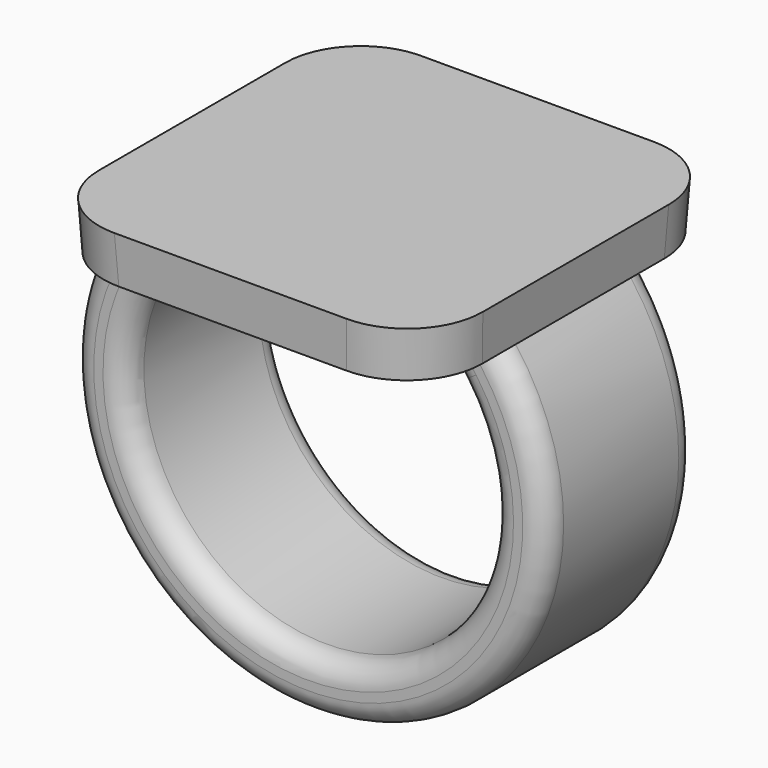
from build123d import *

# Parameters (mm, degrees)
F0_W          = 25.4
F0_H          = 25.4
F1_DEPTH      = 3.175
F1_TAPER      = -3
F3_W          = 5.08
F3_H          = 12.7
F6_DEPTH      = 6.35
F6_DEPTH_BACK = 6.35
F7_R          = 5.08
F8_R          = 1.524


with BuildPart() as f1:
    # F0 (on Top) → F1 (new body)
    with BuildSketch(Plane.XY):
        Rectangle(F0_W, F0_H)
    extrude(amount=F1_DEPTH, taper=F1_TAPER)

    # F4: sweep along a path in F2
    with BuildLine(Plane.XZ) as f4_path:
        ThreePointArc((-10.16, 0), (0, -23.5582897328), (10.16, 0))
    # F3 (on face) → F4 (sweep)
    with BuildSketch(Plane(origin=(0, 0, 0), x_dir=(1, 0, 0), z_dir=(0, 0, -1))):
        with Locations((-10.16, 0)):
            Rectangle(F3_W, F3_H)
    sweep(path=f4_path.line)

    # F5 (on Front) → F6 (join, two sides)
    with BuildSketch(Plane.XZ) as f6_sk:
        with BuildLine():
            Line((10.0130578512, -2.535746045), (10.16, 0))
            Line((10.16, 0), (7.62, 0))
            ThreePointArc((7.62, 0), (8.9072265211, -1.1822790439), (10.0130578512, -2.535746045))
        make_face()
    extrude(amount=F6_DEPTH)
    extrude(f6_sk.sketch, amount=-F6_DEPTH_BACK)

    # F7
    f7_edges = [f1.edges().sort_by_distance(p)[0] for p in [
        (-12.783197, -12.783197, 1.5875),
        (-12.783197, 12.783197, 1.5875),
        (12.783197, 12.783197, 1.5875),
        (12.783197, -12.783197, 1.5875),
    ]]
    fillet(f7_edges, radius=F7_R)

    # F8
    f8_edges = [f1.edges().sort_by_distance(p)[0] for p in [
        (-1.743325, -6.35, -21.711017),
        (8.907227, -6.35, -1.182279),
        (-1.743325, 6.35, -21.711017),
        (0, 6.35, -25.501344),
        (0, -6.35, -25.501344),
        (8.907227, 6.35, -1.182279),
    ]]
    fillet(f8_edges, radius=F8_R)


solid = f1.part
